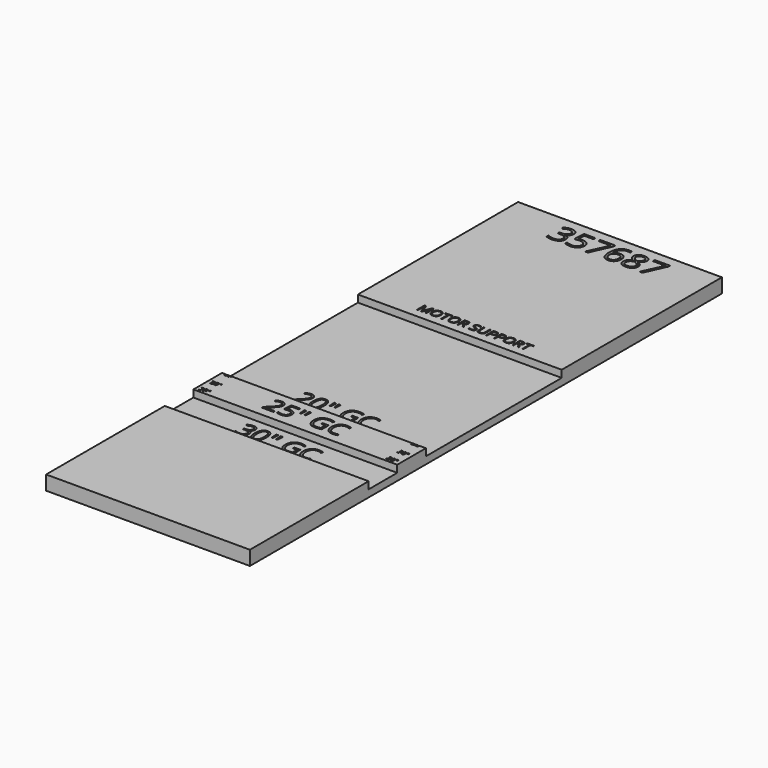
from build123d import *

# Parameters (mm, degrees)
F0_W           = 723.9
F0_H           = 2095.5
F1_DEPTH       = 25.4
F2_W           = 723.9
F2_H           = 127
F2_H_2         = 527.05
F2_H_3         = 711.2
F3_DEPTH       = 25.4
F4_TEXT_SIZE   = 113.0478249656
F4_TEXT_SIZE_2 = 47.4071337117
F4_TEXT_SIZE_3 = 87.5208940771
F5_DEPTH       = 25.4
F5_DEPTH_BACK  = 25.4
F6_TEXT_SIZE   = 22.7675669723
F7_DEPTH       = 25.4
F7_DEPTH_BACK  = 25.4


# Not quite as in the source:
# - Text() gives the source's letters only with a copy of the font that has no kerning and outlines rounded to 1/6400 em; it was checked with that copy


with BuildPart() as f1:
    # F0 (on Top) → F1 (new body)
    with BuildSketch(Plane.XY):
        with Locations((4.8693418503, 561.8504943811)):
            Rectangle(F0_W, F0_H)
    extrude(amount=F1_DEPTH)

    # F2 (on face) → F3 (join)
    with BuildSketch(Plane.XY.offset(25.4)):
        with Locations((4.8693418503, 231.6504943811)):
            Rectangle(F2_W, F2_H)
        with Locations((4.8693418503, -222.3745056189)):
            Rectangle(F2_W, F2_H_2)
        with Locations((4.8693418503, 1254.0004943811)):
            Rectangle(F2_W, F2_H_3)
    extrude(amount=F3_DEPTH)

    # F4 (on face) → F5 (cut, two sides)
    with BuildSketch(Plane.XY.offset(25.4)) as f5_sk:
        with Locations((-171.3279299438, 1493.4318065643)):
            Text('357687', F4_TEXT_SIZE, font='Open Sans', text_align=(TextAlign.LEFT, TextAlign.BOTTOM))
        with Locations((-176.5790991485, 928.9220571518)):
            Text('MOTOR SUPPORT', F4_TEXT_SIZE_2, font='Open Sans', text_align=(TextAlign.LEFT, TextAlign.BOTTOM))
        with Locations((-138.7617159635, 325.4747390747)):
            Text('20" GC', F4_TEXT_SIZE_3, font='Open Sans', text_align=(TextAlign.LEFT, TextAlign.BOTTOM))
        with Locations((-144.4439888, 201.0848224163)):
            Text('25" GC', F4_TEXT_SIZE_3, font='Open Sans', text_align=(TextAlign.LEFT, TextAlign.BOTTOM))
        with Locations((-144.7799950838, 75.9387984872)):
            Text('30" GC', F4_TEXT_SIZE_3, font='Open Sans', text_align=(TextAlign.LEFT, TextAlign.BOTTOM))
    extrude(amount=-F5_DEPTH, mode=Mode.SUBTRACT)
    extrude(f5_sk.sketch, amount=F5_DEPTH_BACK, mode=Mode.SUBTRACT)

    # F6 (on face) → F7 (cut, two sides)
    with BuildSketch(Plane.XY.offset(25.4)) as f7_sk:
        with Locations((319.0148472786, 288.3253097534)):
            Text('25"', F6_TEXT_SIZE, font='Open Sans', text_align=(TextAlign.LEFT, TextAlign.BOTTOM))
        with Locations((318.9071416855, 225.5509197712)):
            Text('30"', F6_TEXT_SIZE, font='Open Sans', text_align=(TextAlign.LEFT, TextAlign.BOTTOM))
        with Locations((319.1503286362, 175.9983599186)):
            Text('20"', F6_TEXT_SIZE, font='Open Sans', text_align=(TextAlign.LEFT, TextAlign.BOTTOM))
        with Locations((-347.0560908318, 288.0974858999)):
            Text('25"', F6_TEXT_SIZE, font='Open Sans', text_align=(TextAlign.LEFT, TextAlign.BOTTOM))
        with Locations((-347.1637964249, 225.3230959177)):
            Text('30"', F6_TEXT_SIZE, font='Open Sans', text_align=(TextAlign.LEFT, TextAlign.BOTTOM))
        with Locations((-346.9206094742, 175.7705360651)):
            Text('20"', F6_TEXT_SIZE, font='Open Sans', text_align=(TextAlign.LEFT, TextAlign.BOTTOM))
    extrude(amount=F7_DEPTH, mode=Mode.SUBTRACT)
    extrude(f7_sk.sketch, amount=-F7_DEPTH_BACK, mode=Mode.SUBTRACT)


solid = f1.part
